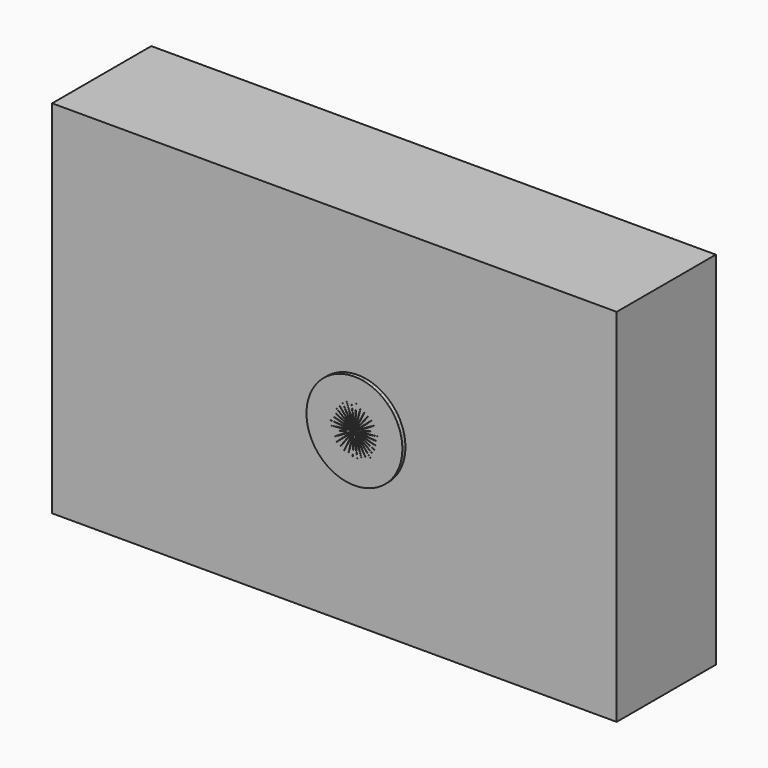
from build123d import *

# Parameters (mm, degrees)
F1_DEPTH = 25
F2_COUNT = 32
F3_DEPTH = 5
F4_W     = 1.956299
F4_H     = 3.493391
F5_DEPTH = 10
F4_W_2   = 22.427575
F4_H_2   = 31.300787
F8_W     = 88.38813
F8_H     = 56.518607
F9_DEPTH = 19.4


with BuildPart() as f1:
    # F0 (on Front) → F1 (new body)
    with BuildSketch(Plane.XZ):
        with BuildLine():
            ThreePointArc((1.19569, 7.404075), (-0.241805, 7.496101), (-1.67038, 7.311623))
            add(Edge.make_bspline(
                [(-1.67038, 7.311623), (-1.564048, 6.631676), (-0.212535, 4.679194), (0.02118, -2.087693), (0.114927, 4.340598), (0.925674, 6.240312), (1.195952, 7.21239), (1.19569, 7.404075)],
                knots=[0, 0, 0, 0, 0.217456, 0.457516, 0.688452, 0.882037, 1, 1, 1, 1], degree=3))
        make_face()
    extrude(amount=F1_DEPTH)

    # F2: F1 ×32 about axis
    f2_axis = Axis((0, 0, 0), (0, -1, 0))


with BuildPart() as f1_1:
    add(f1.part)
    for i in range(1, F2_COUNT):
        add(f1.part.rotate(f2_axis, i * 360 / F2_COUNT))

    # F3 (add): a face of the model
    f3_faces = [f1_1.faces().sort_by_distance(p)[0] for p in [
        (-1.219316, 0, -7.185144),
    ]]
    extrude(f3_faces, amount=F3_DEPTH)


with BuildPart() as f5:
    # F4 (on Front) → F5 (new body)
    with BuildSketch(Plane.XZ):
        with Locations((12.143946, -12.29646)):
            Rectangle(F4_W, F4_H)
    extrude(amount=-F5_DEPTH)


with BuildPart() as f5b:
    # F4 (on Front) → F5, piece 2 (new body)
    with BuildSketch(Plane.XZ):
        with Locations((-0.39733, -1.536814)):
            Rectangle(F4_W_2, F4_H_2)
    extrude(amount=-F5_DEPTH)


with BuildPart() as f9:
    # F8 (on offset) → F9 (new body)
    with BuildSketch(Plane.XZ.offset(24.4)):
        with Locations((-3.61022, 1.120411)):
            Rectangle(F8_W, F8_H)
    extrude(amount=-F9_DEPTH)


solid = Compound([f1_1.part, f5b.part, f9.part])
